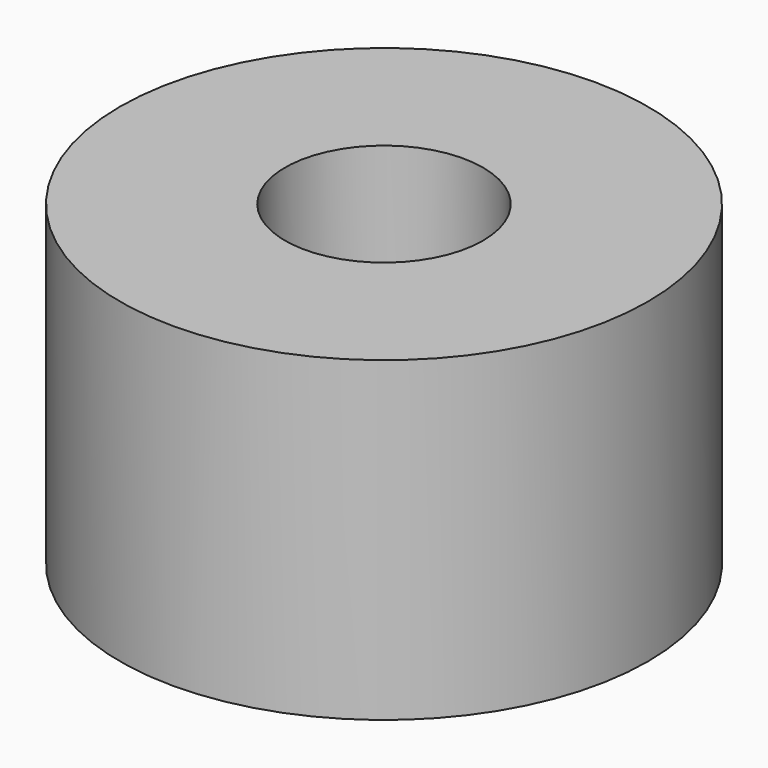
from build123d import *

# Parameters (mm, degrees)
F0_R         = 10
F1_DEPTH     = 12
F2_R         = 1.8
F3_DEPTH     = 5
F4_R         = 3.75
F5_DEPTH     = 25
F6_TEXT_SIZE = 6.846750468
F7_DEPTH     = 0.5
F8_TEXT_SIZE = 5.8611892458
F9_DEPTH     = 0.5


# Not quite as in the source:
# - Text() gives the source's letters only with a copy of the font that has no kerning and outlines rounded to 1/6400 em; it was checked with that copy


with BuildPart() as f1:
    # F0 (on Top) → F1 (new body)
    with BuildSketch(Plane.XY):
        Circle(F0_R)
    extrude(amount=F1_DEPTH)

    # F2 (on face) → F3 (cut)
    with BuildSketch(Plane(origin=(0, 0, 0), x_dir=(1, 0, 0), z_dir=(0, 0, -1))):
        Circle(F2_R)
    extrude(amount=-F3_DEPTH, mode=Mode.SUBTRACT)

    # F4 (on face) → F5 (cut)
    with BuildSketch(Plane(origin=(0, 0, 5), x_dir=(1, 0, 0), z_dir=(0, 0, -1))):
        Circle(F4_R)
    extrude(amount=-F5_DEPTH, mode=Mode.SUBTRACT)

    # F6 (on face) → F7 (cut)
    with BuildSketch(Plane(origin=(0, 0, 0), x_dir=(1, 0, 0), z_dir=(0, 0, -1))):
        with Locations((-6.1342885944, 2.4405239293)):
            Text('v0.1', F6_TEXT_SIZE, font='Open Sans', text_align=(TextAlign.LEFT, TextAlign.BOTTOM))
    extrude(amount=-F7_DEPTH, mode=Mode.SUBTRACT)

    # F8 (on face) → F9 (cut)
    with BuildSketch(Plane(origin=(0, 0, 0), x_dir=(1, 0, 0), z_dir=(0, 0, -1))):
        with Locations((-7.2465080574, -6.3478696898)):
            Text('MM2', F8_TEXT_SIZE, font='Open Sans', text_align=(TextAlign.LEFT, TextAlign.BOTTOM))
    extrude(amount=-F9_DEPTH, mode=Mode.SUBTRACT)


solid = f1.part
